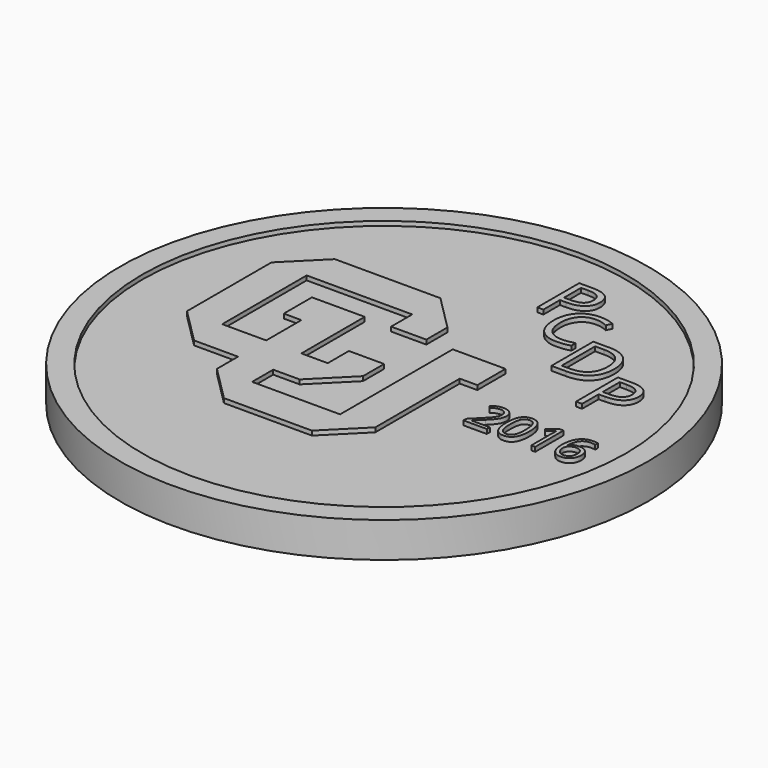
from build123d import *

# Parameters (mm, degrees)
F0_R           = 38.1
F1_DEPTH       = 3.81
F2_R           = 38.1
F2_R_2         = 34.925
F2_TEXT_SIZE   = 10.5833333333
F2_TEXT_SIZE_2 = 7.1690073953
F3_DEPTH       = 0.635
F4_R           = 38.1
F4_R_2         = 34.925
F4_TEXT_SIZE   = 10.5833333333
F5_DEPTH       = 0.635


# Not quite as in the source:
# - Text() gives the source's letters only with a copy of the font that has no kerning and outlines rounded to 1/6400 em; it was checked with that copy


with BuildPart() as f1:
    # F0 (on Top) → F1 (new body)
    with BuildSketch(Plane.XY):
        Circle(F0_R)
    extrude(amount=F1_DEPTH)

    # F2 (on face) → F3 (join)
    with BuildSketch(Plane.XY.offset(3.81)):
        Circle(F2_R)
        Circle(F2_R_2, mode=Mode.SUBTRACT)
        with Locations((13.97, 11.43)):
            Text('D', F2_TEXT_SIZE, font='Open Sans', text_align=(TextAlign.LEFT, TextAlign.BOTTOM))
        with Locations((21.59, 6.35)):
            Text('P', F2_TEXT_SIZE, font='Open Sans', text_align=(TextAlign.LEFT, TextAlign.BOTTOM))
        with Locations((7.62, 16.51)):
            Text('C', F2_TEXT_SIZE, font='Open Sans', text_align=(TextAlign.LEFT, TextAlign.BOTTOM))
        with Locations((3.81, 21.59)):
            Text('P', F2_TEXT_SIZE, font='Open Sans', text_align=(TextAlign.LEFT, TextAlign.BOTTOM))
        with Locations((15.24, -5.1616853246)):
            Text('2016', F2_TEXT_SIZE_2, font='Open Sans', text_align=(TextAlign.LEFT, TextAlign.BOTTOM))
        Polygon((0, -3.81), (0, 0), (-5.08, 0), (-5.08, -3.81), (-8.89, -3.81), (-8.89, 7.62), (-16.51, 7.62), (-16.51, 2.54), (-13.97, 2.54), (-13.97, -3.81), (-20.32, -3.81), (-20.32, 11.43), (-5.08, 11.43), (-5.08, 7.62), (0, 7.62), (0, 11.43), (-5.08, 16.51), (-20.32, 16.51), (-25.4, 11.43), (-25.4, -3.81), (-20.32, -8.89), (-13.97, -8.89), (-13.97, -12.7), (-8.89, -17.78), (3.81, -17.78), (8.89, -12.7), (8.89, 2.54), (11.43, 2.54), (11.43, 7.62), (3.81, 7.62), (3.81, -12.7), (-8.89, -12.7), (-8.89, -8.89), (-5.08, -8.89), align=None)
    extrude(amount=F3_DEPTH)

    # F4 (on face) → F5 (join)
    with BuildSketch(Plane(origin=(0, 0, 0), x_dir=(1, 0, 0), z_dir=(0, 0, -1))):
        Circle(F4_R)
        Circle(F4_R_2, mode=Mode.SUBTRACT)
        with BuildLine():
            Line((-28.251147458, 15.24), (-22.9502561211, 15.24))
            Line((-22.9502561211, 15.24), (-18.9469797359, 15.24))
            Line((-18.9469797359, 15.24), (-22.5166694212, 18.8096896854))
            ThreePointArc((-22.5166694212, 18.8096896854), (-25.6892494631, 17.5153556566), (-28.251147458, 15.24))
        make_face()
        with BuildLine():
            Line((-21.4380400896, 18.9882962107), (-17.6897438789, 15.24))
            Line((-17.6897438789, 15.24), (-14.859, 12.4092561211))
            Line((-14.859, 12.4092561211), (-14.859, 17.4575596876))
            ThreePointArc((-14.859, 17.4575596876), (-18.0175852303, 18.7856801802), (-21.4380400896, 18.9882962107))
        make_face()
        with BuildLine():
            Line((-13.97, 11.5202561211), (-13.97, 8.89))
            Line((-13.97, 8.89), (-13.97, 7.5169797359))
            Line((-13.97, 7.5169797359), (-10.4003103146, 11.0866694212))
            ThreePointArc((-10.4003103146, 11.0866694212), (-11.6946443434, 14.2592494631), (-13.97, 16.821147458))
            Line((-13.97, 16.821147458), (-13.97, 11.5202561211))
        make_face()
        with BuildLine():
            Line((-10.2217037893, 10.0080400896), (-13.97, 6.2597438789))
            Line((-13.97, 6.2597438789), (-16.8007438789, 3.429))
            Line((-16.8007438789, 3.429), (-11.7524403124, 3.429))
            ThreePointArc((-11.7524403124, 3.429), (-10.4243198198, 6.5875852303), (-10.2217037893, 10.0080400896))
        make_face()
        with BuildLine():
            Line((-12.388852542, 2.54), (-17.6897438789, 2.54))
            Line((-17.6897438789, 2.54), (-21.6930202641, 2.54))
            Line((-21.6930202641, 2.54), (-18.1233305788, -1.0296896854))
            ThreePointArc((-18.1233305788, -1.0296896854), (-14.9507505369, 0.2646443434), (-12.388852542, 2.54))
        make_face()
        with BuildLine():
            Line((-19.2019599104, -1.2082962107), (-22.9502561211, 2.54))
            Line((-22.9502561211, 2.54), (-25.781, 5.3707438789))
            Line((-25.781, 5.3707438789), (-25.781, 0.3224403124))
            ThreePointArc((-25.781, 0.3224403124), (-22.6224147697, -1.0056801802), (-19.2019599104, -1.2082962107))
        make_face()
        with BuildLine():
            Line((-26.67, 0.958852542), (-26.67, 6.2597438789))
            Line((-26.67, 6.2597438789), (-26.67, 10.2630202641))
            Line((-26.67, 10.2630202641), (-30.2396896854, 6.6933305788))
            ThreePointArc((-30.2396896854, 6.6933305788), (-28.9453556566, 3.5207505369), (-26.67, 0.958852542))
        make_face()
        with BuildLine():
            Line((-23.8392561211, 14.351), (-28.8875596876, 14.351))
            ThreePointArc((-28.8875596876, 14.351), (-30.2156801802, 11.1924147697), (-30.4182962107, 7.7719599104))
            Line((-30.4182962107, 7.7719599104), (-26.67, 11.5202561211))
            Line((-26.67, 11.5202561211), (-23.8392561211, 14.351))
        make_face()
        with Locations((-7.62, 10.16)):
            Text('Lauren', F4_TEXT_SIZE, font='Open Sans', text_align=(TextAlign.LEFT, TextAlign.BOTTOM))
        with Locations((-5.08, 1.27)):
            Text('Darling', F4_TEXT_SIZE, font='Open Sans', text_align=(TextAlign.LEFT, TextAlign.BOTTOM))
        with Locations((-29.289375, -17.145)):
            Text('For Science!', F4_TEXT_SIZE, font='Open Sans', text_align=(TextAlign.LEFT, TextAlign.BOTTOM))
    extrude(amount=F5_DEPTH)


solid = f1.part
